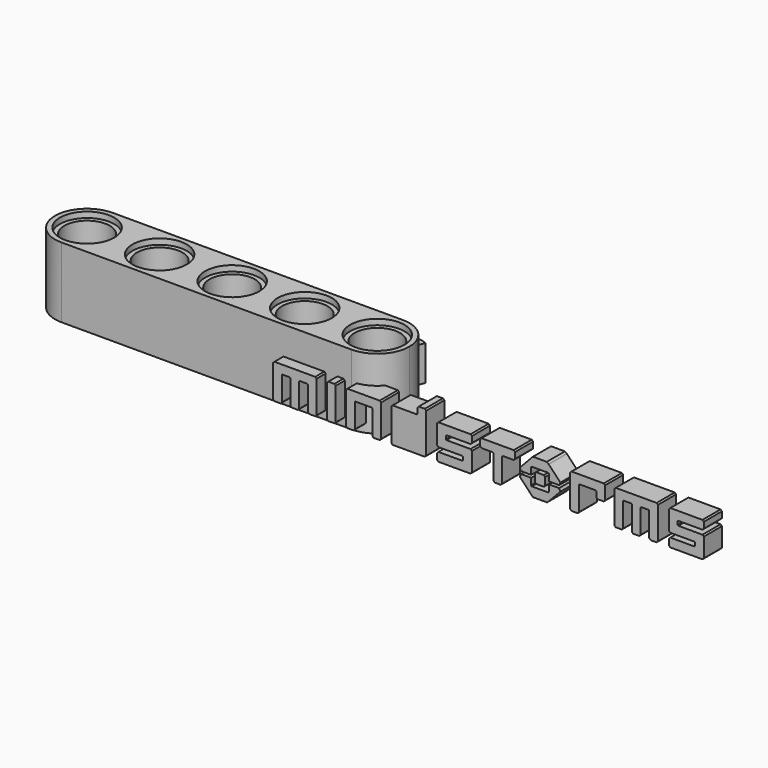
from build123d import *

# Parameters (mm, degrees)
F0_R         = 3.048
F0_R_2       = 2.54
F1_DEPTH     = 3.937
F2_R         = 3.0417071759
F3_DEPTH     = 0.635
F4_R         = 3.048
F5_DEPTH     = 0.635
F6_TEXT_SIZE = 7.5637000716
F7_DEPTH     = 3.937
F8_SIZE2     = 0.50799
F8_SIZE      = 0.50799
F9_SIZE2     = 0.50799
F9_SIZE      = 0.50799
F11_DEPTH    = 1.27
F12_SCALE    = 2


# Not quite as in the source:
# - a fillet or chamfer is up to 0.001 mm smaller than in the source, because OpenCascade refuses the exact size
# - Text() gives the source's letters only with a copy of the font that has no kerning and outlines rounded to 1/6400 em; it was checked with that copy


with BuildPart() as f1:
    # F0 (on Top) → F1 (new body, symmetric)
    with BuildSketch(Plane.XY):
        with BuildLine():
            ThreePointArc((-40.9946195992, 14.3710068385), (-42.0464330806, 16.9103092103), (-44.5857354524, 17.9621226917))
            ThreePointArc((-44.5857354524, 17.9621226917), (-48.1768513056, 14.3710068385), (-44.5857354524, 10.7798909853))
            ThreePointArc((-44.5857354524, 10.7798909853), (-42.0464330806, 11.8317044667), (-40.9946195992, 14.3710068385))
        make_face()
        with Locations((-44.5857354524, 14.3710068385)):
            Circle(F0_R, mode=Mode.SUBTRACT)
        with BuildLine():
            ThreePointArc((-49.1226195992, 14.3710068385), (-50.1744330806, 16.9103092103), (-52.7137354524, 17.9621226917))
            ThreePointArc((-52.7137354524, 17.9621226917), (-56.3048513056, 14.3710068385), (-52.7137354524, 10.7798909853))
            ThreePointArc((-52.7137354524, 10.7798909853), (-50.1744330806, 11.8317044667), (-49.1226195992, 14.3710068385))
        make_face()
        with Locations((-52.7137354524, 14.3710068385)):
            Circle(F0_R, mode=Mode.SUBTRACT)
        with BuildLine():
            ThreePointArc((-32.8666195992, 14.3710068385), (-33.9184330806, 16.9103092103), (-36.4577354524, 17.9621226917))
            ThreePointArc((-36.4577354524, 17.9621226917), (-40.0488513056, 14.3710068385), (-36.4577354524, 10.7798909853))
            ThreePointArc((-36.4577354524, 10.7798909853), (-33.9184330806, 11.8317044667), (-32.8666195992, 14.3710068385))
        make_face()
        with Locations((-36.4577354524, 14.3710068385)):
            Circle(F0_R, mode=Mode.SUBTRACT)
        with BuildLine():
            ThreePointArc((-24.7386195992, 14.3710068385), (-25.7904330806, 16.9103092103), (-28.3297354524, 17.9621226917))
            ThreePointArc((-28.3297354524, 17.9621226917), (-31.9208513056, 14.3710068385), (-28.3297354524, 10.7798909853))
            ThreePointArc((-28.3297354524, 10.7798909853), (-25.7904330806, 11.8317044667), (-24.7386195992, 14.3710068385))
        make_face()
        with Locations((-28.3297354524, 14.3710068385)):
            Circle(F0_R, mode=Mode.SUBTRACT)
        with BuildLine():
            ThreePointArc((-60.8417354524, 10.7798909853), (-58.3024330806, 11.8317044667), (-57.2506195992, 14.3710068385))
            ThreePointArc((-57.2506195992, 14.3710068385), (-58.3024330806, 16.9103092103), (-60.8417354524, 17.9621226917))
            ThreePointArc((-60.8417354524, 17.9621226917), (-64.4328513056, 14.3710068385), (-60.8417354524, 10.7798909853))
        make_face()
        with Locations((-60.8417354524, 14.3710068385)):
            Circle(F0_R, mode=Mode.SUBTRACT)
        with Locations((-44.5857354524, 14.3710068385)):
            Circle(F0_R)
        with Locations((-44.5857354524, 14.3710068385)):
            Circle(F0_R_2, mode=Mode.SUBTRACT)
        with Locations((-36.4577354524, 14.3710068385)):
            Circle(F0_R)
        with Locations((-36.4577354524, 14.3710068385)):
            Circle(F0_R_2, mode=Mode.SUBTRACT)
        with Locations((-52.7137354524, 14.3710068385)):
            Circle(F0_R)
        with Locations((-52.7137354524, 14.3710068385)):
            Circle(F0_R_2, mode=Mode.SUBTRACT)
        with Locations((-28.3297354524, 14.3710068385)):
            Circle(F0_R)
        with Locations((-28.3297354524, 14.3710068385)):
            Circle(F0_R_2, mode=Mode.SUBTRACT)
        with Locations((-60.8417354524, 14.3710068385)):
            Circle(F0_R)
        with Locations((-60.8417354524, 14.3710068385)):
            Circle(F0_R_2, mode=Mode.SUBTRACT)
        with BuildLine():
            ThreePointArc((-60.8417354524, 17.9621226917), (-58.3024330806, 16.9103092103), (-57.2506195992, 14.3710068385))
            ThreePointArc((-57.2506195992, 14.3710068385), (-58.3024330806, 11.8317044667), (-60.8417354524, 10.7798909853))
            Line((-60.8417354524, 10.7798909853), (-52.7137354524, 10.7798909853))
            ThreePointArc((-52.7137354524, 10.7798909853), (-56.3048513056, 14.3710068385), (-52.7137354524, 17.9621226917))
            Line((-52.7137354524, 17.9621226917), (-60.8417354524, 17.9621226917))
        make_face()
        with BuildLine():
            Line((-44.5857354524, 17.9621226917), (-52.7137354524, 17.9621226917))
            ThreePointArc((-52.7137354524, 17.9621226917), (-50.1744330806, 16.9103092103), (-49.1226195992, 14.3710068385))
            ThreePointArc((-49.1226195992, 14.3710068385), (-50.1744330806, 11.8317044667), (-52.7137354524, 10.7798909853))
            Line((-52.7137354524, 10.7798909853), (-44.5857354524, 10.7798909853))
            ThreePointArc((-44.5857354524, 10.7798909853), (-48.1768513056, 14.3710068385), (-44.5857354524, 17.9621226917))
        make_face()
        with BuildLine():
            Line((-28.3297354524, 17.9621226917), (-36.4577354524, 17.9621226917))
            ThreePointArc((-36.4577354524, 17.9621226917), (-33.9184330806, 16.9103092103), (-32.8666195992, 14.3710068385))
            ThreePointArc((-32.8666195992, 14.3710068385), (-33.9184330806, 11.8317044667), (-36.4577354524, 10.7798909853))
            Line((-36.4577354524, 10.7798909853), (-28.3297354524, 10.7798909853))
            ThreePointArc((-28.3297354524, 10.7798909853), (-31.9208513056, 14.3710068385), (-28.3297354524, 17.9621226917))
        make_face()
        with BuildLine():
            Line((-36.4577354524, 17.9621226917), (-44.5857354524, 17.9621226917))
            ThreePointArc((-44.5857354524, 17.9621226917), (-42.0464330806, 16.9103092103), (-40.9946195992, 14.3710068385))
            ThreePointArc((-40.9946195992, 14.3710068385), (-42.0464330806, 11.8317044667), (-44.5857354524, 10.7798909853))
            Line((-44.5857354524, 10.7798909853), (-36.4577354524, 10.7798909853))
            ThreePointArc((-36.4577354524, 10.7798909853), (-40.0488513056, 14.3710068385), (-36.4577354524, 17.9621226917))
        make_face()
    extrude(amount=F1_DEPTH, both=True)

    # F2 (on face) → F3 (cut)
    with BuildSketch(Plane.XY.offset(3.937)):
        with Locations((-28.3297354524, 14.3710068385)):
            Circle(F2_R)
        with Locations((-36.4577354524, 14.3710068385)):
            Circle(F2_R)
        with Locations((-44.5857354524, 14.3710068385)):
            Circle(F2_R)
        with Locations((-52.7137354524, 14.3710068385)):
            Circle(F2_R)
        with Locations((-60.8417354524, 14.3710068385)):
            Circle(F2_R)
    extrude(amount=-F3_DEPTH, mode=Mode.SUBTRACT)

    # F4 (on face) → F5 (cut)
    with BuildSketch(Plane(origin=(0, 0, -3.937), x_dir=(1, 0, 0), z_dir=(0, 0, -1))):
        with Locations((-60.8417354524, -14.3710068385)):
            Circle(F4_R)
        with Locations((-52.7137354524, -14.3710068385)):
            Circle(F4_R)
        with Locations((-44.5857354524, -14.3710068385)):
            Circle(F4_R)
        with Locations((-36.4577354524, -14.3710068385)):
            Circle(F4_R)
        with Locations((-28.3297354524, -14.3710068385)):
            Circle(F4_R)
    extrude(amount=-F5_DEPTH, mode=Mode.SUBTRACT)

    # F6 (on Top) → F7 (join)
    with BuildSketch(Plane.XY):
        with Locations((-60.9262157232, 17.7584644407)):
            Text('bazmarc', F6_TEXT_SIZE, font='Open Sans', font_style=FontStyle.BOLD, text_align=(TextAlign.LEFT, TextAlign.BOTTOM))
    extrude(amount=-F7_DEPTH)

    # F8 (size 0.508 and 0.508 in the source; OpenCascade refuses exactly that, so slightly less here)
    f8_edges = [f1.edges().sort_by_distance(p)[0] for p in [
        (-38.997735, 14.371007, -3.302),
    ]]
    chamfer(f8_edges, length=F8_SIZE, length2=F8_SIZE2)

    # F9 (size 0.508 and 0.508 in the source; OpenCascade refuses exactly that, so slightly less here)
    f9_edges = [f1.edges().sort_by_distance(p)[0] for p in [
        (-47.125735, 14.371007, -3.302),
        (-55.253735, 14.371007, -3.302),
        (-63.381735, 14.371007, -3.302),
        (-30.869735, 14.371007, -3.302),
    ]]
    chamfer(f9_edges, length=F9_SIZE, length2=F9_SIZE2)


with BuildPart() as f11:
    # F10 (on face) → F11 (new body)
    with BuildSketch(Plane.XZ.offset(-10.7798909853)):
        Polygon((6.4595248, 0.7751572), (6.436106, 0.7751572), (4.6791372, 0.7751572), (4.654296, 0.7751572), (4.581271, 0.7035038), (4.581271, 0.678688), (4.581271, -1.075563), (4.581271, -1.0989818), (4.654296, -1.1706352), (4.6791372, -1.1706352), (4.9712626, -1.1706352), (4.9947068, -1.1706352), (5.0677318, -1.0989818), (5.0677318, -1.075563), (5.0677318, 0.2418588), (5.0677318, 0.2487422), (5.1049428, 0.2886964), (5.1173126, 0.2886964), (5.9978798, 0.2886964), (6.0089288, 0.2886964), (6.0461398, 0.254254), (6.0461398, 0.2418588), (6.0461398, -0.0185928), (6.0461398, -0.042037), (6.1191648, -0.115062), (6.1439806, -0.115062), (6.436106, -0.115062), (6.4595248, -0.115062), (6.5326006, -0.042037), (6.5326006, -0.0185928), (6.5326006, 0.678688), (6.5326006, 0.7035038), align=None)
    extrude(amount=F11_DEPTH)


with BuildPart() as f11b:
    # F10 (on face) → F11, piece 2 (new body)
    with BuildSketch(Plane.XZ.offset(-10.7798909853)):
        Polygon((-9.7007172, 0.7751572), (-9.724136, 0.7751572), (-11.9634508, 0.7751572), (-11.9882666, 0.7751572), (-12.0612916, 0.7035038), (-12.0612916, 0.678688), (-12.0612916, -1.075563), (-12.0612916, -1.0989818), (-11.9882666, -1.1706352), (-11.9634508, -1.1706352), (-11.6713, -1.1706352), (-11.6478812, -1.1706352), (-11.5734592, -1.0989818), (-11.5734592, -1.075563), (-11.5734592, 0.2418588), (-11.5734592, 0.254254), (-11.5376452, 0.2886964), (-11.5252246, 0.2886964), (-11.135233, 0.2886964), (-11.1242348, 0.2886964), (-11.0870238, 0.254254), (-11.0870238, 0.2418588), (-11.0870238, -1.075563), (-11.0870238, -1.0989818), (-11.0139734, -1.1706352), (-10.989183, -1.1706352), (-10.6970322, -1.1706352), (-10.6736134, -1.1706352), (-10.600563, -1.0989818), (-10.600563, -1.075563), (-10.600563, 0.2418588), (-10.600563, 0.2487422), (-10.564749, 0.2886964), (-10.5523284, 0.2886964), (-10.1623622, 0.2886964), (-10.1513386, 0.2886964), (-10.1141276, 0.254254), (-10.1141276, 0.2418588), (-10.1141276, -1.075563), (-10.1141276, -1.0989818), (-10.0410772, -1.1706352), (-10.0162868, -1.1706352), (-9.724136, -1.1706352), (-9.7007172, -1.1706352), (-9.6262952, -1.0989818), (-9.6262952, -1.075563), (-9.6262952, 0.678688), (-9.6262952, 0.7035038), align=None)
    extrude(amount=F11_DEPTH)


with BuildPart() as f11c:
    # F10 (on face) → F11, piece 3 (new body)
    with BuildSketch(Plane.XZ.offset(-10.7798909853)):
        Polygon((-6.0930028, 0.7751572), (-6.1164216, 0.7751572), (-7.8748128, 0.7751572), (-7.8996032, 0.7751572), (-7.9726282, 0.7035038), (-7.9726282, 0.678688), (-7.9726282, -1.075563), (-7.9726282, -1.0989818), (-7.8996032, -1.1706352), (-7.8748128, -1.1706352), (-7.584059, -1.1706352), (-7.5606402, -1.1706352), (-7.4861928, -1.0989818), (-7.4861928, -1.075563), (-7.4861928, 0.2418588), (-7.4861928, 0.2487422), (-7.4490072, 0.2886964), (-7.4365866, 0.2886964), (-6.5546478, 0.2886964), (-6.5435988, 0.2886964), (-6.5064132, 0.254254), (-6.5064132, 0.2418588), (-6.5064132, -1.075563), (-6.5064132, -1.0989818), (-6.4333628, -1.1706352), (-6.4085724, -1.1706352), (-6.1164216, -1.1706352), (-6.0930028, -1.1706352), (-6.0199778, -1.0989818), (-6.0199778, -1.075563), (-6.0199778, 0.678688), (-6.0199778, 0.7035038), align=None)
    extrude(amount=F11_DEPTH)


with BuildPart() as f11d:
    # F10 (on face) → F11, piece 4 (new body)
    with BuildSketch(Plane.XZ.offset(-10.7798909853)):
        Polygon((-3.5642804, 1.195451), (-3.5877246, 1.195451), (-3.8785038, 1.195451), (-3.9033196, 1.195451), (-3.9763446, 1.122426), (-3.9763446, 1.0976102), (-3.9763446, 0.8247634), (-3.9763446, 0.8123682), (-4.0135556, 0.7751572), (-4.0245538, 0.7751572), (-5.3460904, 0.7751572), (-5.3709062, 0.7751572), (-5.442585, 0.7035038), (-5.442585, 0.678688), (-5.442585, -1.075563), (-5.442585, -1.0989818), (-5.3709062, -1.1706352), (-5.3460904, -1.1706352), (-3.5877246, -1.1706352), (-3.5642804, -1.1706352), (-3.4898838, -1.0989818), (-3.4898838, -1.075563), (-3.4898838, 1.0976102), (-3.4898838, 1.122426), align=None)
        Polygon((-3.9763446, 0.2418588), (-3.9763446, -0.6373368), (-3.9763446, -0.6483604), (-4.0135556, -0.6841998), (-4.0245538, -0.6841998), (-4.9078896, -0.6841998), (-4.9203102, -0.6841998), (-4.9560988, -0.6483604), (-4.9560988, -0.6373368), (-4.9560988, 0.2418588), (-4.9560988, 0.254254), (-4.9203102, 0.2886964), (-4.9078896, 0.2886964), (-4.0245538, 0.2886964), (-4.0135556, 0.2886964), (-3.9763446, 0.254254), align=None, mode=Mode.SUBTRACT)
        Polygon((-3.9763446, -0.6483604), (-3.9763446, -0.6373368), (-3.9763446, 0.2418588), (-3.9763446, 0.254254), (-4.0135556, 0.2886964), (-4.0245538, 0.2886964), (-4.9078896, 0.2886964), (-4.9203102, 0.2886964), (-4.9560988, 0.254254), (-4.9560988, 0.2418588), (-4.9560988, -0.6373368), (-4.9560988, -0.6483604), (-4.9203102, -0.6841998), (-4.9078896, -0.6841998), (-4.0245538, -0.6841998), (-4.0135556, -0.6841998), align=None)
    extrude(amount=F11_DEPTH)


with BuildPart() as f11e:
    # F10 (on face) → F11, piece 5 (new body)
    with BuildSketch(Plane.XZ.offset(-10.7798909853)):
        Polygon((10.6005376, 0.0930148), (10.6005376, 0.2418588), (10.6005376, 0.254254), (10.6350054, 0.2886964), (10.6474006, 0.2886964), (11.9634254, 0.2886964), (11.9868696, 0.2886964), (12.0612662, 0.3631184), (12.0612662, 0.3865372), (12.0612662, 0.678688), (12.0612662, 0.7035038), (11.9868696, 0.7751572), (11.9634254, 0.7751572), (10.210546, 0.7751572), (10.1857556, 0.7751572), (10.1141022, 0.7035038), (10.1141022, 0.678688), (10.1141022, -0.345186), (10.1141022, -0.3700018), (10.1857556, -0.4444238), (10.210546, -0.4444238), (11.530711, -0.4444238), (11.5362482, -0.4444238), (11.5734338, -0.4774946), (11.5734338, -0.4898898), (11.5734338, -0.6373368), (11.5734338, -0.6483604), (11.5348512, -0.6828028), (11.5293394, -0.6841998), (10.210546, -0.6841998), (10.1857556, -0.6841998), (10.1141022, -0.7585964), (10.1141022, -0.7834122), (10.1141022, -1.075563), (10.1141022, -1.0989818), (10.1857556, -1.1706352), (10.210546, -1.1706352), (11.9634254, -1.1706352), (11.9868696, -1.1706352), (12.0612662, -1.0989818), (12.0612662, -1.075563), (12.0612662, -0.0530606), (12.0612662, -0.0282448), (11.9868696, 0.0434086), (11.9634254, 0.0434086), (10.6487722, 0.0434086), (10.636377, 0.0434086), (10.6005376, 0.0806196), align=None)
    extrude(amount=F11_DEPTH)


with BuildPart() as f11f:
    # F10 (on face) → F11, piece 6 (new body)
    with BuildSketch(Plane.XZ.offset(-10.7798909853)):
        Polygon((-2.3902162, 0.0930148), (-2.3902162, 0.2418588), (-2.3902162, 0.254254), (-2.3557738, 0.2886964), (-2.3433532, 0.2886964), (-1.0273284, 0.2886964), (-1.0039096, 0.2886964), (-0.929513, 0.3631184), (-0.929513, 0.3865372), (-0.929513, 0.678688), (-0.929513, 0.7035038), (-1.0039096, 0.7751572), (-1.0273284, 0.7751572), (-2.7802078, 0.7751572), (-2.8049982, 0.7751572), (-2.8766516, 0.7035038), (-2.8766516, 0.678688), (-2.8766516, -0.345186), (-2.8766516, -0.3700018), (-2.8049982, -0.4444238), (-2.7802078, -0.4444238), (-1.4586712, -0.4444238), (-1.4531594, -0.4444238), (-1.41732, -0.4774946), (-1.41732, -0.4898898), (-1.41732, -0.6373368), (-1.41732, -0.6483604), (-1.455928, -0.6828028), (-1.4614144, -0.6841998), (-2.7802078, -0.6841998), (-2.8049982, -0.6841998), (-2.8766516, -0.7585964), (-2.8766516, -0.7834122), (-2.8766516, -1.075563), (-2.8766516, -1.0989818), (-2.8049982, -1.1706352), (-2.7802078, -1.1706352), (-1.0273284, -1.1706352), (-1.0039096, -1.1706352), (-0.929513, -1.0989818), (-0.929513, -1.075563), (-0.929513, -0.0530606), (-0.929513, -0.0282448), (-1.0039096, 0.0434086), (-1.0273284, 0.0434086), (-2.3419816, 0.0434086), (-2.3543768, 0.0434086), (-2.3902162, 0.0806196), align=None)
    extrude(amount=F11_DEPTH)


with BuildPart() as f11g:
    # F10 (on face) → F11, piece 7 (new body)
    with BuildSketch(Plane.XZ.offset(-10.7798909853)):
        Polygon((1.4131544, 0.7751572), (1.3897356, 0.7751572), (-0.3631184, 0.7751572), (-0.3879088, 0.7751572), (-0.4609846, 0.7035038), (-0.4609846, 0.678688), (-0.4609846, 0.3865372), (-0.4609846, 0.3631184), (-0.3879088, 0.2886964), (-0.3631184, 0.2886964), (0.2280666, 0.2886964), (0.2390648, 0.2886964), (0.2749296, 0.2501138), (0.2763012, 0.2432304), (0.2763012, -1.075563), (0.2763012, -1.0989818), (0.3479292, -1.1706352), (0.372745, -1.1706352), (0.6648704, -1.1706352), (0.68834, -1.1706352), (0.7627366, -1.0989818), (0.7627366, -1.075563), (0.7627366, 0.2418588), (0.7627366, 0.254254), (0.798576, 0.2886964), (0.8109712, 0.2886964), (1.3897356, 0.2886964), (1.4131544, 0.2886964), (1.4862048, 0.3631184), (1.4862048, 0.3865372), (1.4862048, 0.678688), (1.4862048, 0.7035038), align=None)
    extrude(amount=F11_DEPTH)


with BuildPart() as f11h:
    # F10 (on face) → F11, piece 8 (new body)
    with BuildSketch(Plane.XZ.offset(-10.7798909853)):
        Polygon((9.4181676, 0.7751572), (9.3947488, 0.7751572), (7.156831, 0.7751572), (7.1320406, 0.7751572), (7.0589648, 0.7035038), (7.0589648, 0.678688), (7.0589648, -1.075563), (7.0589648, -1.0989818), (7.1320406, -1.1706352), (7.156831, -1.1706352), (7.4475848, -1.1706352), (7.471029, -1.1706352), (7.545451, -1.0989818), (7.545451, -1.075563), (7.545451, 0.2418588), (7.545451, 0.254254), (7.581265, 0.2886964), (7.5936856, 0.2886964), (7.9836518, 0.2886964), (7.9946754, 0.2886964), (8.0319118, 0.254254), (8.0319118, 0.2418588), (8.0319118, -1.075563), (8.0319118, -1.0989818), (8.1049368, -1.1706352), (8.1297272, -1.1706352), (8.4218526, -1.1706352), (8.4452968, -1.1706352), (8.5197188, -1.0989818), (8.5197188, -1.075563), (8.5197188, 0.2418588), (8.5197188, 0.254254), (8.5555328, 0.2886964), (8.5679534, 0.2886964), (8.957945, 0.2886964), (8.9689432, 0.2886964), (9.0061796, 0.254254), (9.0061796, 0.2418588), (9.0061796, -1.075563), (9.0061796, -1.0989818), (9.0791792, -1.1706352), (9.103995, -1.1706352), (9.3947488, -1.1706352), (9.4181676, -1.1706352), (9.492615, -1.0989818), (9.492615, -1.075563), (9.492615, 0.678688), (9.492615, 0.7035038), align=None)
    extrude(amount=F11_DEPTH)


with BuildPart() as f11i:
    # F10 (on face) → F11, piece 9 (new body)
    with BuildSketch(Plane.XZ.offset(-10.7798909853)):
        Polygon((-8.5555582, -1.0989818), (-8.5555582, -1.075563), (-8.5555582, 0.678688), (-8.5555582, 0.7035038), (-8.6299802, 0.7751572), (-8.653399, 0.7751572), (-8.9455498, 0.7751572), (-8.9703402, 0.7751572), (-9.0433906, 0.7035038), (-9.0433906, 0.678688), (-9.0433906, -1.075563), (-9.0433906, -1.0989818), (-8.9703402, -1.1706352), (-8.9455498, -1.1706352), (-8.653399, -1.1706352), (-8.6299802, -1.1706352), align=None)
    extrude(amount=F11_DEPTH)


with BuildPart() as f11j:
    # F10 (on face) → F11, piece 10 (new body)
    with BuildSketch(Plane.XZ.offset(-10.7798909853)):
        Polygon((3.9391082, -0.270764), (3.3920176, -0.270764), (3.3920176, -0.6359652), (3.3920176, -0.6469888), (3.3548066, -0.6828028), (3.3438084, -0.6828028), (2.439797, -0.6828028), (2.4274018, -0.6828028), (2.3915878, -0.6428486), (2.3915878, -0.6373368), (2.3929594, -0.270764), (1.8431256, -0.270764), (1.8197068, -0.270764), (1.7549368, -0.4237482), (1.765935, -0.4347718), (2.386076, -1.0893298), (2.4122634, -1.1155172), (2.4907748, -1.195451), (2.5266142, -1.195451), (3.2583628, -1.195451), (3.2831532, -1.195451), (3.3589722, -1.1265408), (3.3837626, -1.1044936), (4.019042, -0.4347718), (4.0300656, -0.4223512), (3.9584122, -0.270764), align=None)
    extrude(amount=F11_DEPTH)


with BuildPart() as f11k:
    # F10 (on face) → F11, piece 11 (new body)
    with BuildSketch(Plane.XZ.offset(-10.7798909853)):
        Polygon((3.3920176, 0.2390902), (3.3934146, -0.1233424), (3.9404798, -0.124714), (3.9597838, -0.124714), (4.0300656, 0.0282448), (4.019042, 0.0392684), (3.3837626, 0.7090156), (3.3617154, 0.7324344), (3.2666178, 0.8013446), (3.2583628, 0.8013446), (2.5266142, 0.8013446), (2.4907748, 0.8013446), (2.4122634, 0.7200392), (2.386076, 0.6924802), (1.765935, 0.0392684), (1.7549368, 0.0296418), (1.8210784, -0.124714), (1.8431256, -0.124714), (2.3929594, -0.124714), (2.3915878, 0.2404618), (2.3915878, 0.2473706), (2.4287734, 0.2873248), (2.441194, 0.2873248), (3.3438084, 0.2873248), (3.3548066, 0.2873248), (3.3920176, 0.2514854), align=None)
    extrude(amount=F11_DEPTH)


with BuildPart() as f11l:
    # F10 (on face) → F11, piece 12 (new body)
    with BuildSketch(Plane.XZ.offset(-10.7798909853)):
        Polygon((3.0805882, 0.0957834), (2.698877, 0.0957834), (2.6740866, 0.0957834), (2.5996392, 0.0213614), (2.5996392, -0.004826), (2.5996392, -0.3865372), (2.5996392, -0.409956), (2.6740866, -0.4830064), (2.698877, -0.4830064), (3.0805882, -0.4830064), (3.105404, -0.4830064), (3.179826, -0.409956), (3.179826, -0.3865372), (3.179826, -0.004826), (3.179826, 0.0213614), (3.105404, 0.0957834), align=None)
    extrude(amount=F11_DEPTH)


with BuildPart() as f11k_1:
    # F12: moved
    add(f11k.part.scale(F12_SCALE).moved(Location((-11.9868696, -9.5098909853, -0.7751572))))


with BuildPart() as f11_1:
    # F12: moved
    add(f11.part.scale(F12_SCALE).moved(Location((-11.9868696, -9.5098909853, -0.7751572))))


with BuildPart() as f11e_1:
    # F12: moved
    add(f11e.part.scale(F12_SCALE).moved(Location((-11.9868696, -9.5098909853, -0.7751572))))


with BuildPart() as f11f_1:
    # F12: moved
    add(f11f.part.scale(F12_SCALE).moved(Location((-11.9868696, -9.5098909853, -0.7751572))))


with BuildPart() as f11d_1:
    # F12: moved
    add(f11d.part.scale(F12_SCALE).moved(Location((-11.9868696, -9.5098909853, -0.7751572))))


with BuildPart() as f11g_1:
    # F12: moved
    add(f11g.part.scale(F12_SCALE).moved(Location((-11.9868696, -9.5098909853, -0.7751572))))


with BuildPart() as f11c_1:
    # F12: moved
    add(f11c.part.scale(F12_SCALE).moved(Location((-11.9868696, -9.5098909853, -0.7751572))))


with BuildPart() as f11h_1:
    # F12: moved
    add(f11h.part.scale(F12_SCALE).moved(Location((-11.9868696, -9.5098909853, -0.7751572))))


with BuildPart() as f11b_1:
    # F12: moved
    add(f11b.part.scale(F12_SCALE).moved(Location((-11.9868696, -9.5098909853, -0.7751572))))


with BuildPart() as f11i_1:
    # F12: moved
    add(f11i.part.scale(F12_SCALE).moved(Location((-11.9868696, -9.5098909853, -0.7751572))))


with BuildPart() as f11j_1:
    # F12: moved
    add(f11j.part.scale(F12_SCALE).moved(Location((-11.9868696, -9.5098909853, -0.7751572))))


with BuildPart() as f11l_1:
    # F12: moved
    add(f11l.part.scale(F12_SCALE).moved(Location((-11.9868696, -9.5098909853, -0.7751572))))


solid = Compound([f1.part, f11k_1.part, f11_1.part, f11e_1.part, f11f_1.part, f11d_1.part, f11g_1.part, f11c_1.part, f11h_1.part, f11b_1.part, f11i_1.part, f11j_1.part, f11l_1.part])
